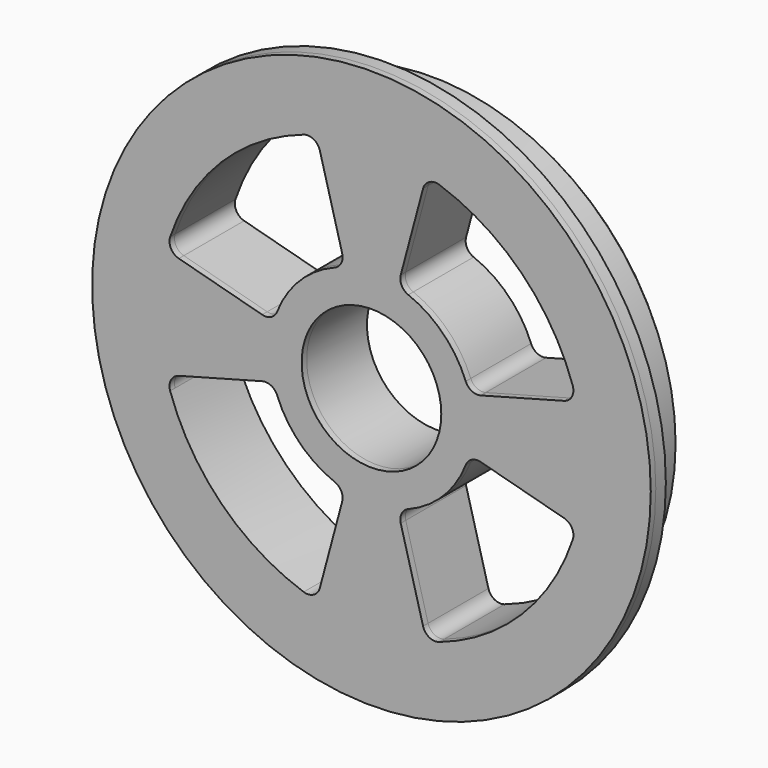
from build123d import *

# Parameters (mm, degrees)
F0_R     = 38.8
F0_R_2   = 11.1125
F1_DEPTH = 12
F2_R     = 44.45
F2_R_2   = 38.8
F3_DEPTH = 2
F6_DEPTH = 25
F7_R     = 2
F8_SIZE  = 1
F9_DEPTH = 1


with BuildPart() as f1:
    # F0 (on Front) → F1 (new body)
    with BuildSketch(Plane.XZ):
        Circle(F0_R)
        Circle(F0_R_2, mode=Mode.SUBTRACT)
    extrude(amount=F1_DEPTH)

    # F2 (on face) → F3 (join)
    with BuildSketch(Plane.XZ.offset(12)):
        Circle(F2_R)
        Circle(F2_R_2, mode=Mode.SUBTRACT)
    extrude(amount=-F3_DEPTH)

    # F5 (on face) → F6 (cut)
    with BuildSketch(Plane.XZ.offset(12)):
        with BuildLine():
            ThreePointArc((8.7480837245, -32.6482929286), (23.9002092041, -23.9002092041), (32.6482929286, -8.7480837245))
            Line((32.6482929286, -8.7480837245), (15.5634798761, -4.1702218642))
            ThreePointArc((15.5634798761, -4.1702218642), (11.3932580119, -11.3932580119), (4.1702218642, -15.5634798761))
            Line((4.1702218642, -15.5634798761), (8.7480837245, -32.6482929286))
        make_face()
        with BuildLine():
            ThreePointArc((-32.6482929286, -8.7480837245), (-23.9002092041, -23.9002092041), (-8.7480837245, -32.6482929286))
            Line((-8.7480837245, -32.6482929286), (-4.1702218642, -15.5634798761))
            ThreePointArc((-4.1702218642, -15.5634798761), (-11.3932580119, -11.3932580119), (-15.5634798761, -4.1702218642))
            Line((-15.5634798761, -4.1702218642), (-32.6482929286, -8.7480837245))
        make_face()
        with BuildLine():
            Line((-4.1702218642, 15.5634798761), (-8.7480837245, 32.6482929286))
            ThreePointArc((-8.7480837245, 32.6482929286), (-23.9002092041, 23.9002092041), (-32.6482929286, 8.7480837245))
            Line((-32.6482929286, 8.7480837245), (-15.5634798761, 4.1702218642))
            ThreePointArc((-15.5634798761, 4.1702218642), (-11.3932580119, 11.3932580119), (-4.1702218642, 15.5634798761))
        make_face()
        with BuildLine():
            Line((15.5634798761, 4.1702218642), (32.6482929286, 8.7480837245))
            ThreePointArc((32.6482929286, 8.7480837245), (23.9002092041, 23.9002092041), (8.7480837245, 32.6482929286))
            Line((8.7480837245, 32.6482929286), (4.1702218642, 15.5634798761))
            ThreePointArc((4.1702218642, 15.5634798761), (11.3932580119, 11.3932580119), (15.5634798761, 4.1702218642))
        make_face()
    extrude(amount=-F6_DEPTH, mode=Mode.SUBTRACT)

    # F7
    f7_edges = [f1.edges().sort_by_distance(p)[0] for p in [
        (-8.748084, -6, -32.648293),
        (-4.170222, -6, -15.56348),
        (-15.56348, -6, -4.170222),
        (-32.648293, -6, -8.748084),
        (4.170222, -6, -15.56348),
        (8.748084, -6, -32.648293),
        (15.56348, -6, -4.170222),
        (32.648293, -6, -8.748084),
        (8.748084, -6, 32.648293),
        (32.648293, -6, 8.748084),
        (15.56348, -6, 4.170222),
        (4.170222, -6, 15.56348),
        (-4.170222, -6, 15.56348),
        (-15.56348, -6, 4.170222),
        (-8.748084, -6, 32.648293),
        (-32.648293, -6, 8.748084),
    ]]
    fillet(f7_edges, radius=F7_R)

    # F8
    f8_edges = [f1.edges().sort_by_distance(p)[0] for p in [
        (-38.8, 0, 0),
    ]]
    chamfer(f8_edges, length=F8_SIZE)

    # F9 (add): a face of the model
    f9_faces = [f1.faces().sort_by_distance(p)[0] for p in [
        (-10.5042580119, -12, -10.5042580119),
    ]]
    extrude(f9_faces, amount=F9_DEPTH)


solid = f1.part
